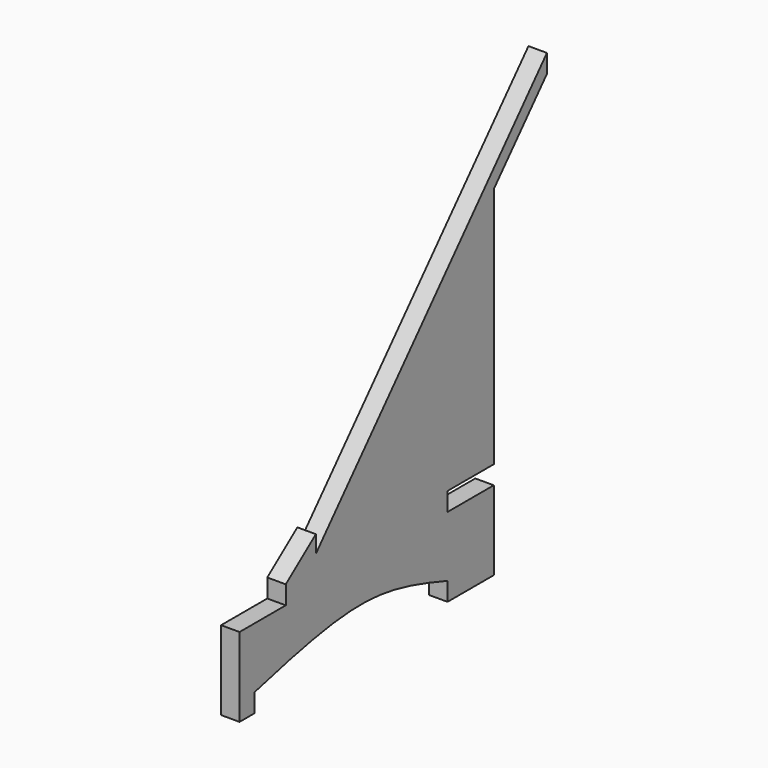
from build123d import *

# Parameters (mm, degrees)
F1_DEPTH = 1.6


# Not quite as in the source:
# - a feature names something its author has since deleted; it is built from what else it names


with BuildPart() as f1:
    # F0 (on Right) → F1 (new body, symmetric)
    with BuildSketch(Plane.YZ):
        with BuildLine():
            Line((-27.5, 0), (-27.5, -3.2))
            Line((-27.5, -3.2), (-24.3, -3.2))
            Line((-24.3, -3.2), (-24.3, 0))
            add(Edge.make_bspline(
                [(-24.3, 0), (-15.858107704, 2.1141811864), (-0.2087572903, 6.0333927878), (11.9158815387, 1.9025152075), (17.5, 0)],
                knots=[0, 0, 0, 0, 0.5394404287, 1, 1, 1, 1], degree=3))
            Line((17.5, 0), (17.5, -3.2))
            Line((17.5, -3.2), (27.5, -3.2))
            Line((27.5, -3.2), (27.5, 0))
            Line((27.5, 0), (27.5, 10.5))
            Line((27.5, 10.5), (17.5, 10.5))
            Line((17.5, 10.5), (17.5, 13.7))
            Line((17.5, 13.7), (27.5, 13.7))
            Line((27.5, 13.7), (27.5, 55.6200032))
            Line((27.5, 55.6200032), (39, 68.5000032))
            Line((39, 68.5000032), (39, 71.7))
            Line((39, 71.7), (-11, 15.7))
            Line((-11, 15.7), (-11, 18.7))
            Line((-11, 18.7), (-17.5, 13.7))
            Line((-17.5, 13.7), (-17.5, 10.5))
            Line((-17.5, 10.5), (-27.5, 10.5))
            Line((-27.5, 10.5), (-27.5, 0))
        make_face()
    extrude(amount=F1_DEPTH, both=True)


solid = f1.part
